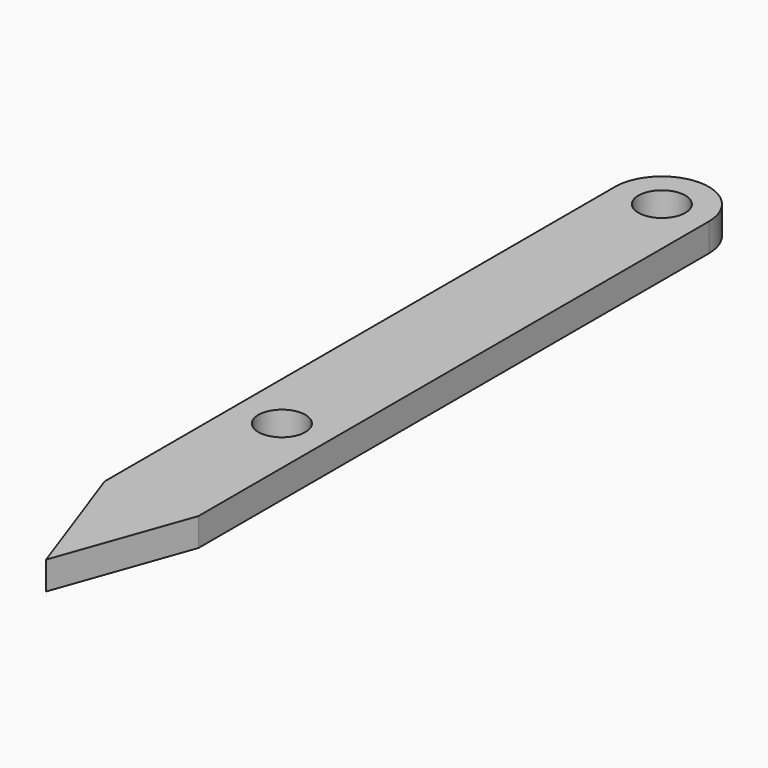
from build123d import *

# Parameters (mm, degrees)
F1_DEPTH = 3.81
F0_R     = 3.175
F2_DEPTH = 3.81


# Not quite as in the source:
# - a feature names something its author has since deleted; it is built from what else it names


with BuildPart() as f1:
    # F0 (on Top) → F1 (new body)
    with BuildSketch(Plane.XY):
        with BuildLine():
            ThreePointArc((-3.175, 52.07), (0, 55.245), (3.175, 52.07))
            Line((3.175, 52.07), (6.35, 52.07))
            ThreePointArc((6.35, 52.07), (0, 58.42), (-6.35, 52.07))
            Line((-6.35, 52.07), (-3.175, 52.07))
        make_face()
    extrude(amount=F1_DEPTH)

    # F0 (on Top) → F2 (join)
    with BuildSketch(Plane.XY):
        Polygon((0, -52.07), (6.35, -34.2291146517), (-6.35, -34.2291146517), align=None)
        with BuildLine():
            Line((6.35, 52.07), (3.175, 52.07))
            ThreePointArc((3.175, 52.07), (0, 48.895), (-3.175, 52.07))
            Line((-3.175, 52.07), (-6.35, 52.07))
            Line((-6.35, 52.07), (-6.35, -34.2291146517))
            Line((-6.35, -34.2291146517), (6.35, -34.2291146517))
            Line((6.35, -34.2291146517), (6.35, 52.07))
        make_face()
        with Locations((0, -12.192)):
            Circle(F0_R, mode=Mode.SUBTRACT)
    extrude(amount=F2_DEPTH)


solid = f1.part
